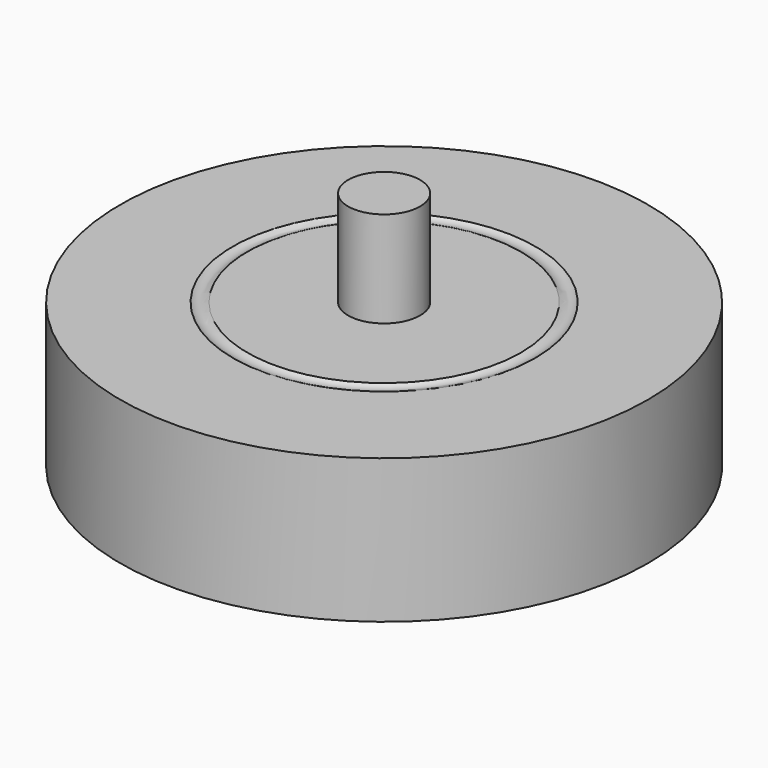
from build123d import *

# Parameters (mm, degrees)
F0_R          = 55
F0_R_2        = 7.5
F1_DEPTH      = 30
F2_T          = -2.5
F4_R          = 2.5
F3_R          = 7.5
F6_DEPTH      = 20
F6_DEPTH_BACK = 5
F7_R          = 10
F7_R_2        = 7.5
F8_DEPTH      = 5.5


with BuildPart() as f1:
    # F0 (on Top) → F1 (new body)
    with BuildSketch(Plane.XY):
        Circle(F0_R)
        Circle(F0_R_2, mode=Mode.SUBTRACT)
    extrude(amount=-F1_DEPTH)

    # F2
    f2_openings = [f1.faces().sort_by_distance(p)[0] for p in [
        (-53.444365, 0, -30),
        (-7.5, 0, -15),
    ]]
    offset(amount=F2_T, openings=f2_openings)

    # F5: sweep along a path in F3
    with BuildLine(Plane.XY) as f5_path:
        CenterArc((0, 0), 30, 0, 360)
    # F4 (on Front) → F5 (sweep, cut)
    with BuildSketch(Plane.XZ):
        with Locations((30, 2)):
            Circle(F4_R)
    sweep(path=f5_path.line, mode=Mode.SUBTRACT)

    # F7 (on face) → F8 (join)
    with BuildSketch(Plane(origin=(0, 0, -2.5), x_dir=(1, 0, 0), z_dir=(0, 0, -1))):
        Circle(F7_R)
        Circle(F7_R_2, mode=Mode.SUBTRACT)
    extrude(amount=F8_DEPTH)


with BuildPart() as f6:
    # F3 (on face) → F6 (new body, two sides)
    with BuildSketch(Plane.XY) as f6_sk:
        Circle(F3_R)
    extrude(amount=F6_DEPTH)
    extrude(f6_sk.sketch, amount=-F6_DEPTH_BACK)


solid = Compound([f1.part, f6.part])
